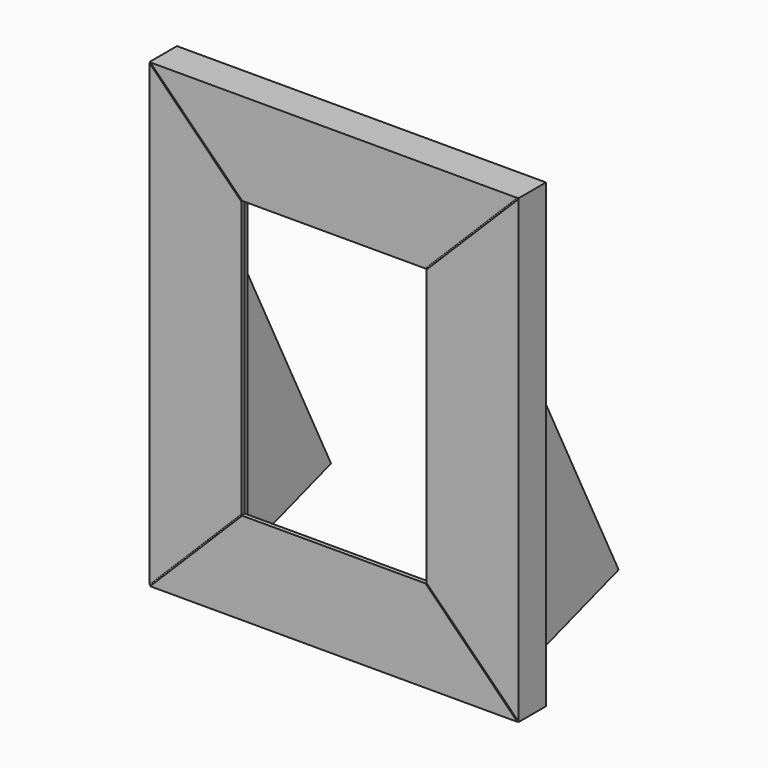
from build123d import *

# Parameters (mm, degrees)
F2_W              = 101.854
F2_H              = 127.3048
F2_W_2            = 51.054
F2_H_2            = 76.5048
F3_DEPTH          = 9.525
F4_W              = 62.992
F4_H              = 111.252
F5_DEPTH          = 8.382
F8_DEPTH          = 3.175
F9_W              = 30.48
F9_H              = 8.0264
F10_DEPTH         = 8.382
F12_DEPTH         = 0.254
F12_COPIES2_COUNT = 2


# Not quite as in the source:
# - a pattern or mirror of a feature is missing from the dataset's text; its kind, count and spacing are read off the source's solid


with BuildPart() as f3:
    # F2 (on Front) → F3 (new body)
    with BuildSketch(Plane.XZ):
        Rectangle(F2_W, F2_H)
        Rectangle(F2_W_2, F2_H_2, mode=Mode.SUBTRACT)
    extrude(amount=F3_DEPTH)

    # F4 (on face) → F5 (cut)
    with BuildSketch(Plane(origin=(0, 0, 0), x_dir=(-1, 0, 0), z_dir=(0, 1, 0))):
        Rectangle(F4_W, F4_H)
    extrude(amount=-F5_DEPTH, mode=Mode.SUBTRACT)

    # F7 (on offset) → F8 (join)
    with BuildSketch(Plane.YZ.offset(38.1)):
        Polygon((37.1396206319, -48.7135574222), (0, 25.9003154933), (0, -60.8499720693), align=None)
    f8 = extrude(amount=F8_DEPTH)

    # F8_copies: F8 across plane
    add(f8.mirror(Plane(origin=(0, 0, 0), x_dir=(0, 0, -1), z_dir=(-1, 0, 0))))

    # F9 (on face) → F10 (cut, through all)
    with BuildSketch(Plane(origin=(0, 0, 0), x_dir=(-1, 0, 0), z_dir=(0, 1, 0))):
        with Locations((0, -59.6392)):
            Rectangle(F9_W, F9_H)
    extrude(amount=-F10_DEPTH, mode=Mode.SUBTRACT)

    # F11 (on face) → F12 (cut)
    with BuildSketch(Plane.XZ.offset(9.525)):
        Polygon((-50.927, 63.3984), (-25.527, 37.9984), (-25.527, 38.2524), (-25.273, 38.2524), (-50.673, 63.6524), (-50.927, 63.6524), align=None)
    f12 = extrude(amount=-F12_DEPTH, mode=Mode.SUBTRACT)

    # F12_copies: F12 across plane
    add(f12.mirror(Plane(origin=(0, 0, 0), x_dir=(0, 0, 1), z_dir=(1, 0, 0))), mode=Mode.SUBTRACT)

    # F12_copies1: F12 across plane
    add(f12.mirror(Plane(origin=(0, 0, 0), x_dir=(-1, 0, 0), z_dir=(0, 0, -1))), mode=Mode.SUBTRACT)

    # F12_copies2: F12 ×2 about axis
    f12_copies2_axis = Axis((0, 0, 0), (0, 1, 0))
    for i in range(1, F12_COPIES2_COUNT):
        add(f12.rotate(f12_copies2_axis, i * 360 / F12_COPIES2_COUNT), mode=Mode.SUBTRACT)


solid = f3.part
